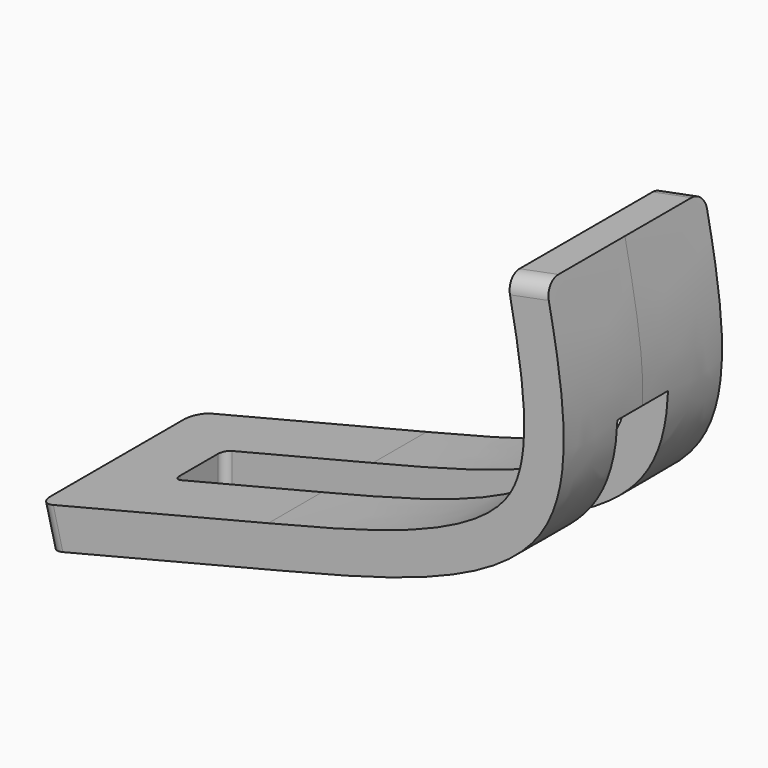
from build123d import *

# Parameters (mm, degrees)
F1_DEPTH      = 12.5
F1_DEPTH_BACK = 12.5
F2_R          = 2
F4_DEPTH      = 25
F4_DEPTH_BACK = 25


# Not quite as in the source:
# - the dataset's text gives a spline's control points without its knots; the knots are read off the source's solid


with BuildPart() as f1:
    # F0 (on Front) → F1 (new body, two sides)
    with BuildSketch(Plane.XZ) as f1_sk:
        with BuildLine():
            Line((-1.2144668808, 4.8502649614), (0, 0))
            add(Edge.make_bspline(
                [(0, 0), (14.0053337055, 3.5068216017), (40.2847665376, 10.0869812236), (35.8928594477, 32.5950939434), (33.8415652514, 43.1077592075)],
                knots=[0, 0, 0, 0, 0.5329389288, 1, 1, 1, 1], degree=3))
            Line((33.8415652514, 43.1077592075), (28.9341160149, 42.1501883266))
            add(Edge.make_bspline(
                [(-1.2144668808, 4.8502649614), (2.0704623451, 5.6727845108), (6.9395130075, 6.8930060669), (12.9580209, 8.6517206422), (17.1378010676, 10.0677938672), (20.8819548221, 11.6030918314), (24.0858702772, 13.2626270815), (26.223316492, 14.7303860036), (27.5858152583, 15.9298585553), (28.2940402512, 16.6843045519), (28.7790865507, 17.2904800643), (29.1028323995, 17.7454757687), (29.3927734629, 18.2085550663), (29.9263537911, 19.1820206107), (30.5546444399, 20.8222293139), (31.0433856174, 23.4947469816), (31.1666131935, 26.6257001867), (30.9497019112, 30.1362027001), (30.2857972333, 35.2092298808), (29.4831057596, 39.3366740929), (28.9341160149, 42.1501883266)],
                knots=[0, 0, 0, 0, 0.125, 0.1875, 0.25, 0.3125, 0.375, 0.4375, 0.46875, 0.5, 0.515625, 0.53125, 0.546875, 0.5625, 0.625, 0.6875, 0.75, 0.8125, 0.875, 1, 1, 1, 1], degree=3))
        make_face()
        Polygon((-29.1015897681, -7.286801285), (0, 0), (-1.2144668808, 4.8502649614), (-30.316056649, -2.4365363237), align=None)
    extrude(amount=F1_DEPTH)
    extrude(f1_sk.sketch, amount=-F1_DEPTH_BACK)

    # F2
    f2_edges = [f1.edges().sort_by_distance(p)[0] for p in [
        (31.387841, -12.5, 42.628974),
        (31.387841, 12.5, 42.628974),
        (-29.708823, -12.5, -4.861669),
        (-29.708823, 12.5, -4.861669),
    ]]
    fillet(f2_edges, radius=F2_R)

    # F3 (on Top) → F4 (cut, two sides)
    with BuildSketch(Plane.XY) as f4_sk:
        with BuildLine():
            Line((-19, -4), (50, -4))
            Line((50, -4), (50, 4))
            Line((50, 4), (-19, 4))
            ThreePointArc((-19, 4), (-19.7071067812, 3.7071067812), (-20, 3))
            Line((-20, 3), (-20, -3))
            ThreePointArc((-20, -3), (-19.7071067812, -3.7071067812), (-19, -4))
        make_face()
    extrude(amount=F4_DEPTH, mode=Mode.SUBTRACT)
    extrude(f4_sk.sketch, amount=-F4_DEPTH_BACK, mode=Mode.SUBTRACT)


solid = f1.part
